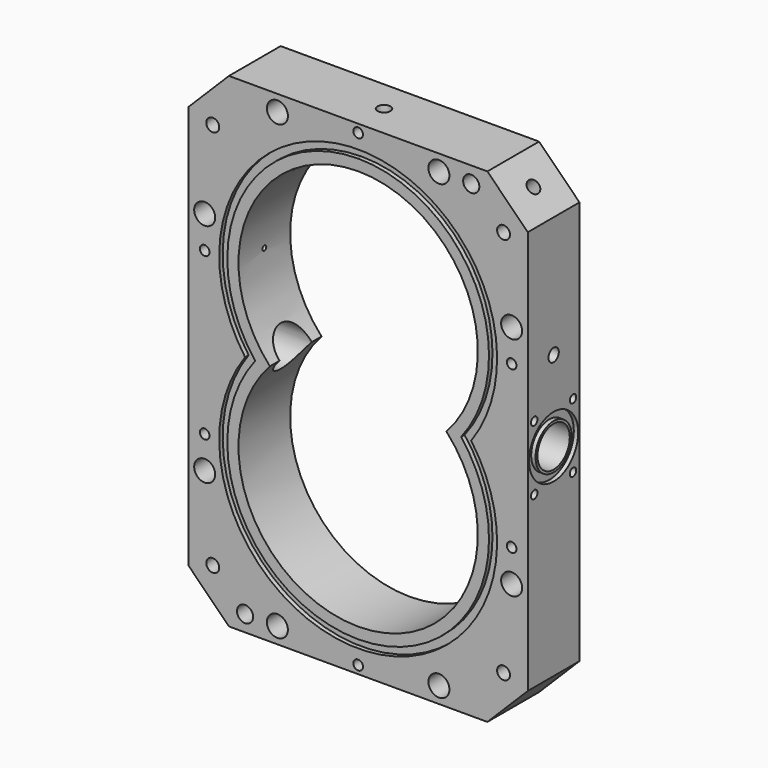
from build123d import *

# Parameters (mm, degrees)
F1_DEPTH  = 20
F2_R      = 12.5
F3_DEPTH  = 210.001
F4_R      = 19
F4_R_2    = 14
F5_DEPTH  = 2.7
F6_R      = 19
F6_R_2    = 14
F7_DEPTH  = 2.7
F9_DEPTH  = 2.7
F11_DEPTH = 2.7
F12_R     = 2.5
F13_DEPTH = 10
F14_R     = 2.5
F15_DEPTH = 10
F16_R     = 6.5
F17_DEPTH = 20
F18_R     = 4.25
F19_DEPTH = 40.0010001
F20_R     = 3
F21_DEPTH = 10
F24_W     = 1.5
F24_H     = 28.0618912584
F26_W     = 24.1605055332
F26_H     = 1.5
F28_R     = 5
F29_DEPTH = 40.0010001
F30_R     = 4
F31_DEPTH = 16


# Not quite as in the source:
# - a pattern or mirror of a feature is missing from the dataset's text; its kind, count and spacing are read off the source's solid


with BuildPart() as f1:
    # F0 (on Front) → F1 (new body, symmetric)
    with BuildSketch(Plane.XZ):
        Polygon((80, 150), (-80, 150), (-105, 125), (-105, -125), (-80, -150), (80, -150), (105, -125), (105, 125), align=None)
        with BuildLine():
            ThreePointArc((-54.6611964743, 0), (0, 124.08), (54.6611964743, 0))
            ThreePointArc((54.6611964743, 0), (0, -124.08), (-54.6611964743, 0))
        make_face(mode=Mode.SUBTRACT)
    extrude(amount=F1_DEPTH, both=True)

    # F2 (on face) → F3 (cut, through all)
    with BuildSketch(Plane.YZ.offset(105)):
        Circle(F2_R)
    extrude(amount=-F3_DEPTH, mode=Mode.SUBTRACT)

    # F4 (on face) → F5 (cut)
    with BuildSketch(Plane.YZ.offset(105)):
        Circle(F4_R)
        Circle(F4_R_2, mode=Mode.SUBTRACT)
    extrude(amount=-F5_DEPTH, mode=Mode.SUBTRACT)

    # F6 (on face) → F7 (cut)
    with BuildSketch(Plane(origin=(-105, 0, 0), x_dir=(0, -1, 0), z_dir=(-1, 0, 0))):
        Circle(F6_R)
        Circle(F6_R_2, mode=Mode.SUBTRACT)
    extrude(amount=-F7_DEPTH, mode=Mode.SUBTRACT)

    # F8 (on face) → F9 (cut)
    with BuildSketch(Plane(origin=(0, 20, 0), x_dir=(-1, 0, 0), z_dir=(0, 1, 0))):
        with BuildLine():
            ThreePointArc((-69.9714227381, 0), (0, -136), (69.9714227381, 0))
            ThreePointArc((69.9714227381, 0), (0, 136), (-69.9714227381, 0))
        make_face()
        with BuildLine():
            ThreePointArc((0, 131), (72.8388632531, 85.4330354331), (63.7259758654, 0))
            ThreePointArc((63.7259758654, 0), (72.8388632531, -85.4330354331), (0, -131))
            ThreePointArc((0, -131), (-72.8388632531, -85.4330354331), (-63.7259758654, 0))
            ThreePointArc((-63.7259758654, 0), (-72.8388632531, 85.4330354331), (0, 131))
        make_face(mode=Mode.SUBTRACT)
    extrude(amount=-F9_DEPTH, mode=Mode.SUBTRACT)

    # F10 (on face) → F11 (cut)
    with BuildSketch(Plane.XZ.offset(20)):
        with BuildLine():
            ThreePointArc((69.9714227381, 0), (0, 136), (-69.9714227381, 0))
            ThreePointArc((-69.9714227381, 0), (0, -136), (69.9714227381, 0))
        make_face()
        with BuildLine():
            ThreePointArc((0, 131), (72.8388632531, 85.4330354331), (63.7259758654, 0))
            ThreePointArc((63.7259758654, 0), (72.8388632531, -85.4330354331), (0, -131))
            ThreePointArc((0, -131), (-72.8388632531, -85.4330354331), (-63.7259758654, 0))
            ThreePointArc((-63.7259758654, 0), (-72.8388632531, 85.4330354331), (0, 131))
        make_face(mode=Mode.SUBTRACT)
    extrude(amount=-F11_DEPTH, mode=Mode.SUBTRACT)

    # F12 (on face) → F13 (cut)
    with BuildSketch(Plane.YZ.offset(105)):
        with Locations((-15, 20)):
            Circle(F12_R)
        with Locations((15, 20)):
            Circle(F12_R)
        with Locations((15, -20)):
            Circle(F12_R)
        with Locations((-15, -20)):
            Circle(F12_R)
    extrude(amount=-F13_DEPTH, mode=Mode.SUBTRACT)

    # F14 (on face) → F15 (cut)
    with BuildSketch(Plane(origin=(-105, 0, 0), x_dir=(0, -1, 0), z_dir=(-1, 0, 0))):
        with Locations((-15, 20)):
            Circle(F14_R)
        with Locations((15, 20)):
            Circle(F14_R)
        with Locations((15, -20)):
            Circle(F14_R)
        with Locations((-15, -20)):
            Circle(F14_R)
    extrude(amount=-F15_DEPTH, mode=Mode.SUBTRACT)

    # F16 (on face) → F17 (cut)
    with BuildSketch(Plane.XZ.offset(20)):
        with Locations((-50, 140)):
            Circle(F16_R)
        with Locations((50, 140)):
            Circle(F16_R)
        with Locations((-50, -140)):
            Circle(F16_R)
        with Locations((50, -140)):
            Circle(F16_R)
        with Locations((95, 70)):
            Circle(F16_R)
        with Locations((95, -70)):
            Circle(F16_R)
        with Locations((-95, 70)):
            Circle(F16_R)
        with Locations((-95, -70)):
            Circle(F16_R)
    extrude(amount=-F17_DEPTH, mode=Mode.SUBTRACT)

    # F18 (on face) → F19 (cut, through all)
    with BuildSketch(Plane.XZ.offset(20)):
        with Locations((-50, 140)):
            Circle(F18_R)
        with Locations((50, 140)):
            Circle(F18_R)
        with Locations((95, 70)):
            Circle(F18_R)
        with Locations((95, -70)):
            Circle(F18_R)
        with Locations((50, -140)):
            Circle(F18_R)
        with Locations((-50, -140)):
            Circle(F18_R)
        with Locations((-95, -70)):
            Circle(F18_R)
        with Locations((-95, 70)):
            Circle(F18_R)
    extrude(amount=-F19_DEPTH, mode=Mode.SUBTRACT)

    # F20 (on face) → F21 (cut)
    with BuildSketch(Plane.XZ.offset(20)):
        with Locations((0, 145)):
            Circle(F20_R)
        with Locations((-95, 50)):
            Circle(F20_R)
        with Locations((-95, -50)):
            Circle(F20_R)
        with Locations((95, -50)):
            Circle(F20_R)
        with Locations((95, 50)):
            Circle(F20_R)
        with Locations((0, -145)):
            Circle(F20_R)
    extrude(amount=-F21_DEPTH, mode=Mode.SUBTRACT)

    # F22 (on Front) → F23 (revolve, cut)
    with BuildSketch(Plane.XZ):
        Polygon((-89.6732207666, 140.3267792334), (-92.5016478914, 137.4983521086), (-85.4305800795, 130.4272842968), (-84.3699199077, 131.4879444685), (-82.6021529548, 133.2557114215), align=None)
        Polygon((-84.3699199077, 131.4879444685), (-85.4305800795, 130.4272842968), (-49.1876475233, 94.1843517405), (-48.1269873515, 95.2450119123), align=None)
    f23 = revolve(axis=Axis((-46.2508239457, 0, 91.2475281629), (0.7071067812, 0, -0.7071067812)), mode=Mode.SUBTRACT)

    # F23_copies: F23 across plane
    add(f23.mirror(Plane(origin=(6e-06, 0, 0), x_dir=(0, 0, 1), z_dir=(1, 0, 0))), mode=Mode.SUBTRACT)

    # F24 (on Front) → F25 (revolve, cut)
    with BuildSketch(Plane.XZ):
        with Locations((0.75, 125.9690543708)):
            Rectangle(F24_W, F24_H)
        Polygon((0, 162.6632596409), (0, 140), (1.5, 140), (4, 140), (4, 162.6632596409), align=None)
    revolve(axis=Axis((0, 0, 81.3316298204), (0, 0, 1)), mode=Mode.SUBTRACT)

    # F26 (on Front) → F27 (revolve, cut)
    with BuildSketch(Plane.XZ):
        with Locations((82.9197472334, 49.25)):
            Rectangle(F26_W, F26_H)
        Polygon((111.5470026106, 50), (95, 50), (95, 48.5), (95, 46), (111.5470026106, 46), align=None)
    f27 = revolve(axis=Axis((9.1493800282, 0, 50), (1, 0, 0)), mode=Mode.SUBTRACT)

    # F27_copies: F27 across plane
    add(f27.mirror(Plane(origin=(1e-06, 0, 0), x_dir=(0, 0, -1), z_dir=(-1, 0, 0))), mode=Mode.SUBTRACT)

    # F28 (on face) → F29 (cut, through all)
    with BuildSketch(Plane.XZ.offset(20)):
        with Locations((70, 140)):
            Circle(F28_R)
        with Locations((-70, -140)):
            Circle(F28_R)
    extrude(amount=-F29_DEPTH, mode=Mode.SUBTRACT)

    # F30 (on face) → F31 (cut)
    with BuildSketch(Plane.XZ.offset(20)):
        with Locations((-90, 120)):
            Circle(F30_R)
        with Locations((90, 120)):
            Circle(F30_R)
        with Locations((90, -120)):
            Circle(F30_R)
        with Locations((-90, -120)):
            Circle(F30_R)
    extrude(amount=-F31_DEPTH, mode=Mode.SUBTRACT)


solid = f1.part
